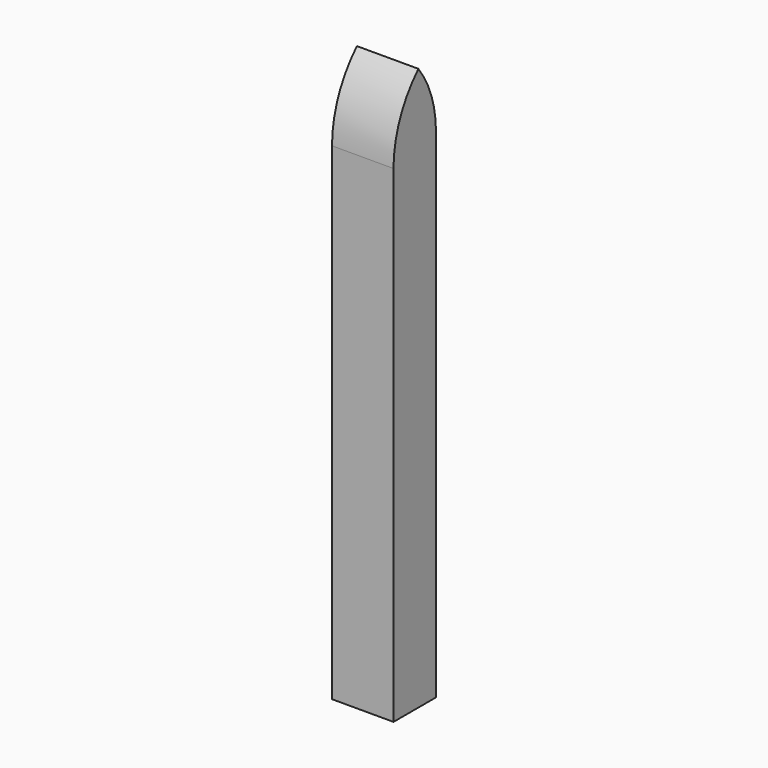
from build123d import *

# Parameters (mm, degrees)
F0_W        = 2.9410525192
F0_H        = 2.54
F1_DEPTH    = 38.1
F2_T1_DEPTH = 68.2618004135
F3_R        = 5.08
F4_T1_DEPTH = 23.6793240582


# Not quite as in the source:
# - a fillet or chamfer that OpenCascade refuses, or shapes differently, is made with other operations: its cross-section is extruded or revolved along the edge and cut away or added


with BuildPart() as f1:
    # F0 (on Top) → F1 (new body)
    with BuildSketch(Plane.XY):
        with Locations((-36.622652784, 43.036242947)):
            Rectangle(F0_W, F0_H)
    extrude(amount=F1_DEPTH)

    # F2: chamfer of 12.7 on 1 edges, made by hand

    # F2_s2 → F2_t1 (cut)
    with BuildSketch(Plane.YZ.offset(-70.7535529908)):
        Polygon((41.766242947, 25.4), (54.466242947, 38.1), (41.766242947, 38.1), align=None)
    extrude(amount=F2_T1_DEPTH, mode=Mode.SUBTRACT)

    # F3
    f3_edges = [f1.edges().sort_by_distance(p)[0] for p in [
        (-36.622653, 41.766243, 25.4),
    ]]
    fillet(f3_edges, radius=F3_R)

    # F4: fillet of radius 5.08 on 1 edges, made by hand

    # F4_s2 → F4_t1 (cut)
    with BuildSketch(Plane.YZ.offset(-48.4623148131)):
        with BuildLine():
            ThreePointArc((43.2541404986, 26.8878975516), (44.0360308613, 25.4270750946), (44.306242947, 23.7923456922))
            Line((44.306242947, 23.7923456922), (44.306242947, 27.94))
            Line((44.306242947, 27.94), (43.2541404986, 26.8878975516))
        make_face()
    extrude(amount=F4_T1_DEPTH, mode=Mode.SUBTRACT)


solid = f1.part
